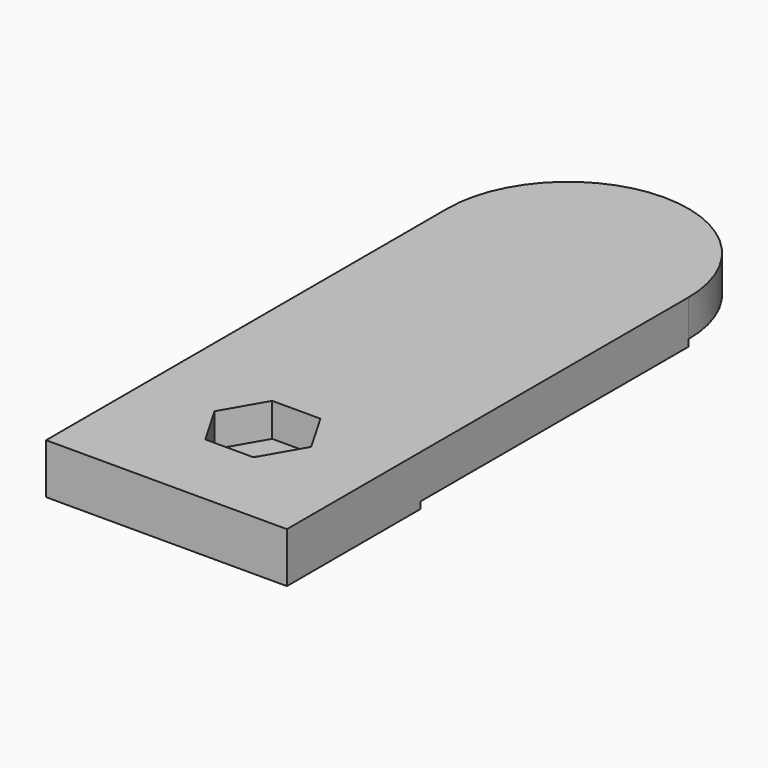
from build123d import *

# Parameters (mm, degrees)
F0_W     = 1.016
F0_H     = 3.556
F0_H_2   = 5.588
F1_DEPTH = 2.794
F2_DEPTH = 0.508
F3_DEPTH = 1.016
F4_R     = 2.54
F5_DEPTH = 1.524
F6_R     = 1.397
F7_DEPTH = 5.334
F9_DEPTH = 2.54


with BuildPart() as f1:
    # F0 (on Top) → F1 (new body)
    with BuildSketch(Plane.XY):
        with BuildLine():
            Line((8.128, 28.956), (9.144, 28.956))
            ThreePointArc((9.144, 28.956), (0, 38.1), (-9.144, 28.956))
            Line((-9.144, 28.956), (-8.128, 28.956))
            Line((-8.128, 28.956), (-2.54, 28.956))
            ThreePointArc((-2.54, 28.956), (0, 31.496), (2.54, 28.956))
            Line((2.54, 28.956), (8.128, 28.956))
        make_face()
        with BuildLine():
            ThreePointArc((-8.128, 24.7669246844), (0, 19.812), (8.128, 24.7669246844))
            Line((8.128, 24.7669246844), (8.128, 28.956))
            Line((8.128, 28.956), (2.54, 28.956))
            ThreePointArc((2.54, 28.956), (0, 26.416), (-2.54, 28.956))
            Line((-2.54, 28.956), (-8.128, 28.956))
            Line((-8.128, 28.956), (-8.128, 24.7669246844))
        make_face()
        with BuildLine():
            Line((8.128, 24.7669246844), (8.128, 9.144))
            Line((8.128, 9.144), (9.144, 9.144))
            Line((9.144, 9.144), (9.144, 28.956))
            ThreePointArc((9.144, 28.956), (8.8863706877, 26.8007385309), (8.128, 24.7669246844))
        make_face()
        with BuildLine():
            Line((8.128, 28.956), (8.128, 24.7669246844))
            ThreePointArc((8.128, 24.7669246844), (8.8863706877, 26.8007385309), (9.144, 28.956))
            Line((9.144, 28.956), (8.128, 28.956))
        make_face()
        with BuildLine():
            ThreePointArc((-2.54, 28.956), (0, 26.416), (2.54, 28.956))
            Line((2.54, 28.956), (-2.54, 28.956))
        make_face()
        with BuildLine():
            Line((-2.54, 28.956), (2.54, 28.956))
            ThreePointArc((2.54, 28.956), (0, 31.496), (-2.54, 28.956))
        make_face()
        with BuildLine():
            ThreePointArc((-9.144, 28.956), (-8.8863706877, 26.8007385309), (-8.128, 24.7669246844))
            Line((-8.128, 24.7669246844), (-8.128, 28.956))
            Line((-8.128, 28.956), (-9.144, 28.956))
        make_face()
        with BuildLine():
            Line((-9.144, 9.144), (-8.128, 9.144))
            Line((-8.128, 9.144), (-8.128, 24.7669246844))
            ThreePointArc((-8.128, 24.7669246844), (-8.8863706877, 26.8007385309), (-9.144, 28.956))
            Line((-9.144, 28.956), (-9.144, 9.144))
        make_face()
        with BuildLine():
            Line((-8.128, 9.144), (8.128, 9.144))
            Line((8.128, 9.144), (8.128, 24.7669246844))
            ThreePointArc((8.128, 24.7669246844), (0, 19.812), (-8.128, 24.7669246844))
            Line((-8.128, 24.7669246844), (-8.128, 9.144))
        make_face()
        Polygon((-8.128, 3.556), (0, 3.556), (8.128, 3.556), (8.128, 9.144), (-8.128, 9.144), align=None)
        with BuildLine():
            ThreePointArc((-2.54, 0), (-1.7960512242, 1.7960512242), (0, 2.54))
            Line((0, 2.54), (0, 3.556))
            Line((0, 3.556), (-8.128, 3.556))
            Line((-8.128, 3.556), (-8.128, 0))
            Line((-8.128, 0), (-2.54, 0))
        make_face()
        with BuildLine():
            Line((0, -9.144), (0, -2.54))
            ThreePointArc((0, -2.54), (-1.7960512242, -1.7960512242), (-2.54, 0))
            Line((-2.54, 0), (-8.128, 0))
            Line((-8.128, 0), (-9.144, 0))
            Line((-9.144, 0), (-9.144, -9.144))
            Line((-9.144, -9.144), (0, -9.144))
        make_face()
        with Locations((-8.636, 1.778)):
            Rectangle(F0_W, F0_H)
        with BuildLine():
            ThreePointArc((0, 2.54), (1.7960512242, 1.7960512242), (2.54, 0))
            Line((2.54, 0), (8.128, 0))
            Line((8.128, 0), (8.128, 3.556))
            Line((8.128, 3.556), (0, 3.556))
            Line((0, 3.556), (0, 2.54))
        make_face()
        with Locations((8.636, 1.778)):
            Rectangle(F0_W, F0_H)
        with BuildLine():
            Line((8.128, 0), (2.54, 0))
            ThreePointArc((2.54, 0), (1.7960512242, -1.7960512242), (0, -2.54))
            Line((0, -2.54), (0, -9.144))
            Line((0, -9.144), (9.144, -9.144))
            Line((9.144, -9.144), (9.144, 0))
            Line((9.144, 0), (8.128, 0))
        make_face()
        with BuildLine():
            ThreePointArc((0, -2.54), (1.7960512242, -1.7960512242), (2.54, 0))
            Line((2.54, 0), (0, 0))
            Line((0, 0), (-2.54, 0))
            ThreePointArc((-2.54, 0), (-1.7960512242, -1.7960512242), (0, -2.54))
        make_face()
        with BuildLine():
            Line((0, 0), (2.54, 0))
            ThreePointArc((2.54, 0), (1.7960512242, 1.7960512242), (0, 2.54))
            ThreePointArc((0, 2.54), (-1.7960512242, 1.7960512242), (-2.54, 0))
            Line((-2.54, 0), (0, 0))
        make_face()
        with Locations((-8.636, 6.35)):
            Rectangle(F0_W, F0_H_2)
        with Locations((8.636, 6.35)):
            Rectangle(F0_W, F0_H_2)
    extrude(amount=F1_DEPTH)

    # F0 (on Top) → F2 (join)
    with BuildSketch(Plane.XY):
        with BuildLine():
            ThreePointArc((-9.144, 28.956), (-8.8863706877, 26.8007385309), (-8.128, 24.7669246844))
            Line((-8.128, 24.7669246844), (-8.128, 28.956))
            Line((-8.128, 28.956), (-9.144, 28.956))
        make_face()
        with BuildLine():
            Line((-9.144, 9.144), (-8.128, 9.144))
            Line((-8.128, 9.144), (-8.128, 24.7669246844))
            ThreePointArc((-8.128, 24.7669246844), (-8.8863706877, 26.8007385309), (-9.144, 28.956))
            Line((-9.144, 28.956), (-9.144, 9.144))
        make_face()
        with BuildLine():
            Line((8.128, 24.7669246844), (8.128, 9.144))
            Line((8.128, 9.144), (9.144, 9.144))
            Line((9.144, 9.144), (9.144, 28.956))
            ThreePointArc((9.144, 28.956), (8.8863706877, 26.8007385309), (8.128, 24.7669246844))
        make_face()
        with BuildLine():
            Line((8.128, 28.956), (8.128, 24.7669246844))
            ThreePointArc((8.128, 24.7669246844), (8.8863706877, 26.8007385309), (9.144, 28.956))
            Line((9.144, 28.956), (8.128, 28.956))
        make_face()
        with Locations((-8.636, 6.35)):
            Rectangle(F0_W, F0_H_2)
        with Locations((8.636, 6.35)):
            Rectangle(F0_W, F0_H_2)
    extrude(amount=-F2_DEPTH)

    # F0 (on Top) → F3 (join)
    with BuildSketch(Plane.XY):
        with BuildLine():
            Line((0, -9.144), (0, -2.54))
            ThreePointArc((0, -2.54), (-1.7960512242, -1.7960512242), (-2.54, 0))
            Line((-2.54, 0), (-8.128, 0))
            Line((-8.128, 0), (-9.144, 0))
            Line((-9.144, 0), (-9.144, -9.144))
            Line((-9.144, -9.144), (0, -9.144))
        make_face()
        with BuildLine():
            ThreePointArc((-2.54, 0), (-1.7960512242, 1.7960512242), (0, 2.54))
            Line((0, 2.54), (0, 3.556))
            Line((0, 3.556), (-8.128, 3.556))
            Line((-8.128, 3.556), (-8.128, 0))
            Line((-8.128, 0), (-2.54, 0))
        make_face()
        with BuildLine():
            ThreePointArc((0, -2.54), (1.7960512242, -1.7960512242), (2.54, 0))
            Line((2.54, 0), (0, 0))
            Line((0, 0), (-2.54, 0))
            ThreePointArc((-2.54, 0), (-1.7960512242, -1.7960512242), (0, -2.54))
        make_face()
        with BuildLine():
            Line((0, 0), (2.54, 0))
            ThreePointArc((2.54, 0), (1.7960512242, 1.7960512242), (0, 2.54))
            ThreePointArc((0, 2.54), (-1.7960512242, 1.7960512242), (-2.54, 0))
            Line((-2.54, 0), (0, 0))
        make_face()
        with BuildLine():
            ThreePointArc((0, 2.54), (1.7960512242, 1.7960512242), (2.54, 0))
            Line((2.54, 0), (8.128, 0))
            Line((8.128, 0), (8.128, 3.556))
            Line((8.128, 3.556), (0, 3.556))
            Line((0, 3.556), (0, 2.54))
        make_face()
        with BuildLine():
            Line((8.128, 0), (2.54, 0))
            ThreePointArc((2.54, 0), (1.7960512242, -1.7960512242), (0, -2.54))
            Line((0, -2.54), (0, -9.144))
            Line((0, -9.144), (9.144, -9.144))
            Line((9.144, -9.144), (9.144, 0))
            Line((9.144, 0), (8.128, 0))
        make_face()
        with Locations((-8.636, 1.778)):
            Rectangle(F0_W, F0_H)
        with Locations((8.636, 1.778)):
            Rectangle(F0_W, F0_H)
    extrude(amount=-F3_DEPTH)

    # F4 (on face) → F5 (join)
    with BuildSketch(Plane(origin=(0, 0, -1.016), x_dir=(1, 0, 0), z_dir=(0, 0, -1))):
        Circle(F4_R)
    extrude(amount=F5_DEPTH)

    # F6 (on face) → F7 (cut, through all)
    with BuildSketch(Plane(origin=(0, 0, -2.54), x_dir=(1, 0, 0), z_dir=(0, 0, -1))):
        Circle(F6_R)
    extrude(amount=-F7_DEPTH, mode=Mode.SUBTRACT)

    # F8 (on face) → F9 (cut)
    with BuildSketch(Plane.XY.offset(2.794)):
        Polygon((-1.8330871047, -3.175), (0, -3.175), (1.8330871047, -3.175), (3.6661742094, 0), (1.8330871047, 3.175), (-1.8330871047, 3.175), (-3.6661742094, 0), align=None)
        with BuildLine():
            ThreePointArc((1.397, 0), (0.9878281733, -0.9878281733), (0, -1.397))
            ThreePointArc((0, -1.397), (-0.9878281733, 0.9878281733), (1.397, 0))
        make_face(mode=Mode.SUBTRACT)
    extrude(amount=-F9_DEPTH, mode=Mode.SUBTRACT)


solid = f1.part
